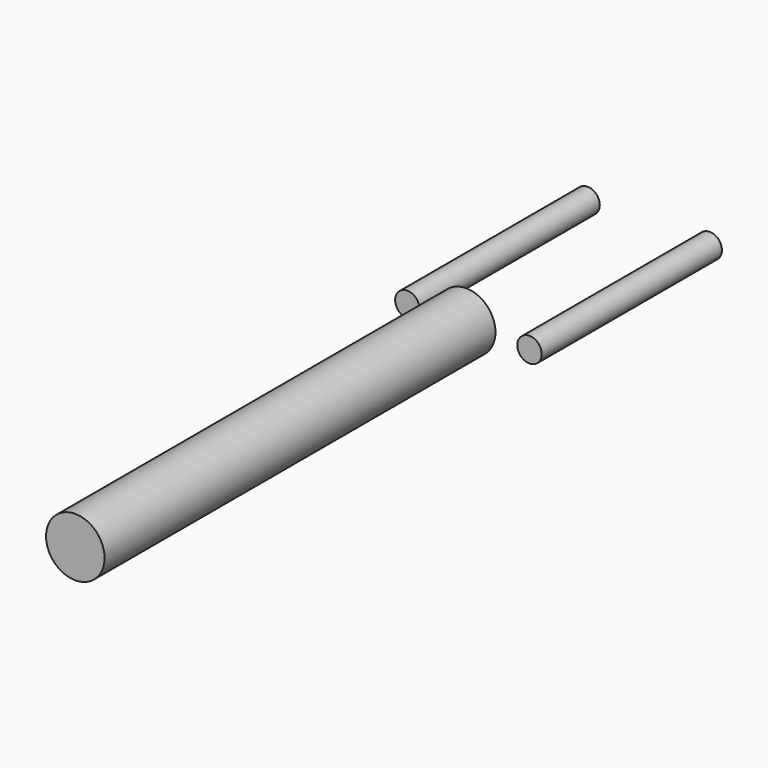
from build123d import *

# Parameters (mm, degrees)
F1_R          = 11.9789339658
F3_DEPTH      = 200
F2_R          = 5
F4_DEPTH      = 48.8475
F4_DEPTH_BACK = 43.35047


# Not quite as in the source:
# - a feature of the source that left no trace in its solid (it failed there, or was rolled back) is left out


with BuildPart() as f3:
    # F1 (on Front) → F3 (new body)
    with BuildSketch(Plane.XZ):
        Circle(F1_R)
    extrude(amount=F3_DEPTH)


with BuildPart() as f4:
    # F2 (on offset) → F4 (new body, two sides)
    with BuildSketch(Plane.XZ.offset(-50)) as f4_sk:
        with Locations((-25, -2.5)):
            Circle(F2_R)
    extrude(amount=F4_DEPTH)
    extrude(f4_sk.sketch, amount=-F4_DEPTH_BACK)


with BuildPart() as f4b:
    # F2 (on offset) → F4, piece 2 (new body, two sides)
    with BuildSketch(Plane.XZ.offset(-50)) as f4_2_sk:
        with Locations((25, -2.5)):
            Circle(F2_R)
    extrude(amount=F4_DEPTH)
    extrude(f4_2_sk.sketch, amount=-F4_DEPTH_BACK)


solid = Compound([f3.part, f4.part, f4b.part])
